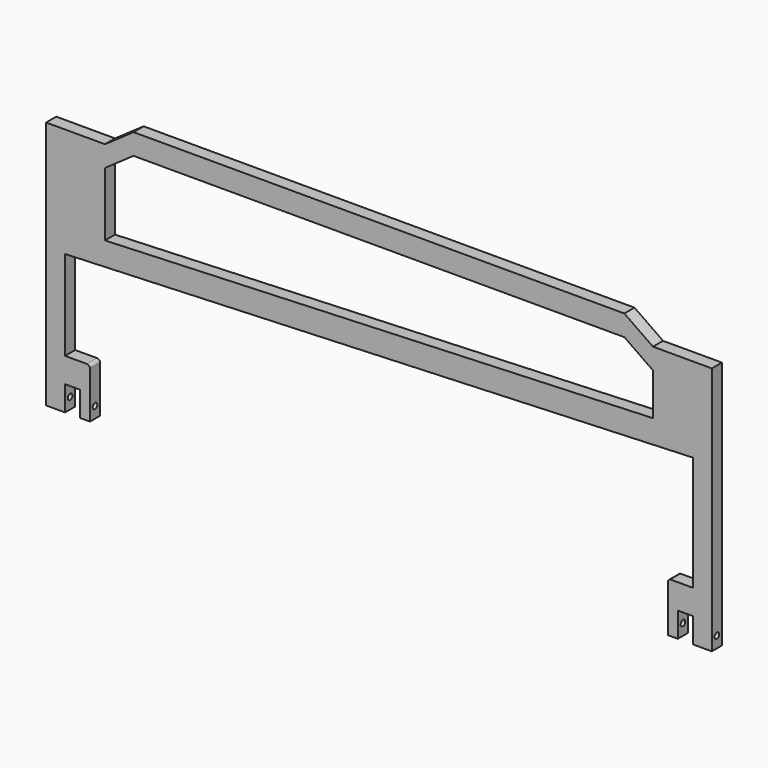
from build123d import *

# Parameters (mm, degrees)
F1_DEPTH = 12.7
F2_R     = 5.8193233161
F3_DEPTH = 1800


# Not quite as in the source:
# - a feature names something its author has since deleted; it is built from what else it names


with BuildPart() as f1:
    # F0 (on Front) → F1 (new body, symmetric)
    with BuildSketch(Plane.XZ):
        with BuildLine():
            Line((492.5543735346, 210), (0, 210))
            Line((0, 210), (-492.5543735346, 210))
            Line((-492.5543735346, 210), (-550, 170))
            Line((-550, 170), (-630, 170))
            Line((-630, 170), (-668.1, 170))
            Line((-668.1, 170), (-668.1, -230))
            Line((-668.1, -230), (-668.1, -330))
            Line((-668.1, -330), (-630, -330))
            Line((-630, -330), (-630, -280))
            Line((-630, -280), (-600, -280))
            Line((-600, -280), (-600, -330))
            Line((-600, -330), (-580, -330))
            Line((-580, -330), (-580, -236.35))
            ThreePointArc((-580, -236.35), (-581.8598719395, -231.8598719395), (-586.35, -230))
            Line((-586.35, -230), (-630, -230))
            Line((-630, -230), (-630, -50))
            Line((-630, -50), (630, 0))
            Line((630, 0), (630, -50))
            Line((630, -50), (630, -230))
            Line((630, -230), (586.35, -230))
            ThreePointArc((586.35, -230), (581.8598719395, -231.8598719395), (580, -236.35))
            Line((580, -236.35), (580, -330))
            Line((580, -330), (600, -330))
            Line((600, -330), (600, -280))
            Line((600, -280), (630, -280))
            Line((630, -280), (630, -330))
            Line((630, -330), (668.1, -330))
            Line((668.1, -330), (668.1, -230))
            Line((668.1, -230), (668.1, 170))
            Line((668.1, 170), (630, 170))
            Line((630, 170), (550, 170))
            Line((550, 170), (492.5543735346, 210))
        make_face()
        Polygon((550, 43.6507936508), (-550, 0), (-550, 128.1044334173), (-492.5543735346, 168.1044334173), (492.5543735346, 168.1044334173), (550, 128.1044334173), align=None, mode=Mode.SUBTRACT)
    extrude(amount=F1_DEPTH, both=True)

    # F2 (on face) → F3 (cut)
    with BuildSketch(Plane.YZ.offset(668.1)):
        with Locations((0, -307.489156723)):
            Circle(F2_R)
    extrude(amount=-F3_DEPTH, mode=Mode.SUBTRACT)


solid = f1.part
